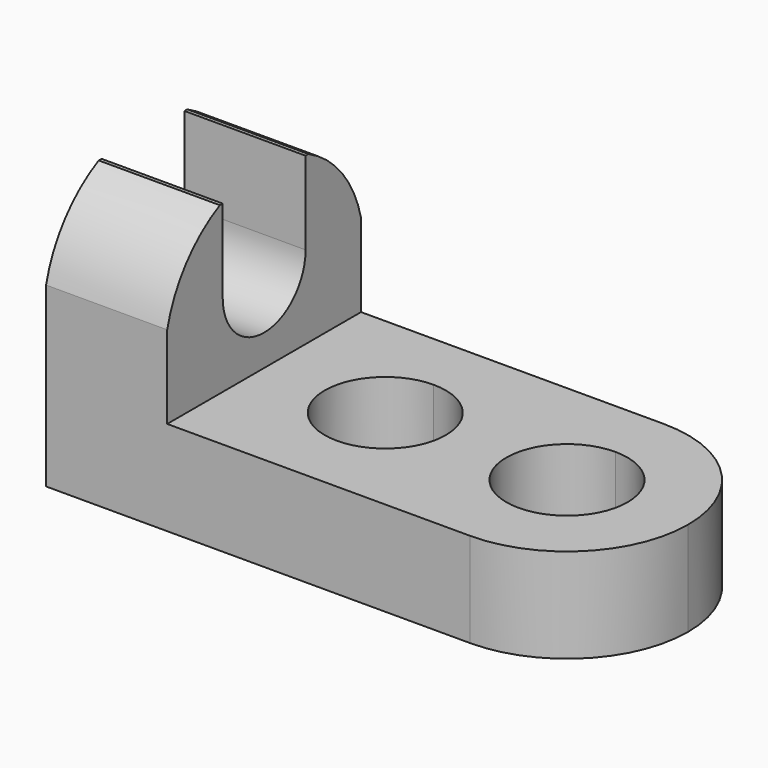
from build123d import *

# Parameters (mm, degrees)
F1_DEPTH = 25.4
F3_DEPTH = 12.701
F5_DEPTH = 9.9016336957


with BuildPart() as f1:
    # F0 (on Front) → F1 (new body)
    with BuildSketch(Plane.XZ):
        Polygon((-29.7019003412, 0), (27.4480996588, 0), (27.4480996588, 9.9006336957), (-17.0019003412, 9.9006336957), (-17.0019003412, 27.2871126172), (-29.7019003412, 27.2871126172), align=None)
    extrude(amount=F1_DEPTH)

    # F2 (on face) → F3 (cut, through all)
    with BuildSketch(Plane.YZ.offset(-17.0019003412)):
        with BuildLine():
            Line((-25.4, 27.2871126172), (-25.4, 18.5938731565))
            ThreePointArc((-25.4, 18.5938731565), (-22.9225497247, 23.7099564427), (-18.5048555567, 27.2871126172))
            Line((-18.5048555567, 27.2871126172), (-25.4, 27.2871126172))
        make_face()
        with BuildLine():
            ThreePointArc((-7.2696510886, 18.5938731565), (-12.7, 24.0242220678), (-18.1303489114, 18.5938731565))
            Line((-18.1303489114, 18.5938731565), (-7.2696510886, 18.5938731565))
        make_face()
        with BuildLine():
            Line((-18.1303489114, 27.2871126172), (-18.1303489114, 18.5938731565))
            ThreePointArc((-18.1303489114, 18.5938731565), (-12.7, 24.0242220678), (-7.2696510886, 18.5938731565))
            Line((-7.2696510886, 18.5938731565), (-7.2696510886, 27.2871126172))
            Line((-7.2696510886, 27.2871126172), (-18.1303489114, 27.2871126172))
        make_face()
        with BuildLine():
            Line((-7.2696510886, 18.5938731565), (-18.1303489114, 18.5938731565))
            ThreePointArc((-18.1303489114, 18.5938731565), (-12.7, 13.1635242451), (-7.2696510886, 18.5938731565))
        make_face()
        with BuildLine():
            ThreePointArc((-6.8951444433, 27.2871126172), (-12.7, 28.6495177359), (-18.5048555567, 27.2871126172))
            Line((-18.5048555567, 27.2871126172), (-18.1303489114, 27.2871126172))
            Line((-18.1303489114, 27.2871126172), (-7.2696510886, 27.2871126172))
            Line((-7.2696510886, 27.2871126172), (-6.8951444433, 27.2871126172))
        make_face()
        with BuildLine():
            Line((0, 27.2871126172), (-6.8951444433, 27.2871126172))
            ThreePointArc((-6.8951444433, 27.2871126172), (-2.4774502753, 23.7099564427), (0, 18.5938731565))
            Line((0, 18.5938731565), (0, 27.2871126172))
        make_face()
    extrude(amount=-F3_DEPTH, mode=Mode.SUBTRACT)

    # F4 (on face) → F5 (cut, through all)
    with BuildSketch(Plane.XY.offset(9.9006336957)):
        with BuildLine():
            Line((14.7480996588, -19.05), (14.7480996588, -6.35))
            ThreePointArc((14.7480996588, -6.35), (8.3980996588, -12.7), (14.7480996588, -19.05))
        make_face()
        with BuildLine():
            ThreePointArc((21.0980996588, -12.7), (19.2382277193, -8.2098719395), (14.7480996588, -6.35))
            Line((14.7480996588, -6.35), (14.7480996588, -19.05))
            ThreePointArc((14.7480996588, -19.05), (19.2382277193, -17.1901280605), (21.0980996588, -12.7))
        make_face()
        with BuildLine():
            Line((-4.3019003412, -19.05), (-4.3019003412, -6.35))
            ThreePointArc((-4.3019003412, -6.35), (-10.6519003412, -12.7), (-4.3019003412, -19.05))
        make_face()
        with BuildLine():
            ThreePointArc((2.0480996588, -12.7), (0.1882277193, -8.2098719395), (-4.3019003412, -6.35))
            Line((-4.3019003412, -6.35), (-4.3019003412, -19.05))
            ThreePointArc((-4.3019003412, -19.05), (0.1882277193, -17.1901280605), (2.0480996588, -12.7))
        make_face()
        with BuildLine():
            Line((27.4480996588, 0), (14.7480996588, 0))
            ThreePointArc((14.7480996588, 0), (23.7283557799, -3.7197438789), (27.4480996588, -12.7))
            Line((27.4480996588, -12.7), (27.4480996588, 0))
        make_face()
        with BuildLine():
            Line((27.4480996588, -25.4), (27.4480996588, -12.7))
            ThreePointArc((27.4480996588, -12.7), (23.7283557799, -21.6802561211), (14.7480996588, -25.4))
            Line((14.7480996588, -25.4), (27.4480996588, -25.4))
        make_face()
    extrude(amount=-F5_DEPTH, mode=Mode.SUBTRACT)


solid = f1.part
